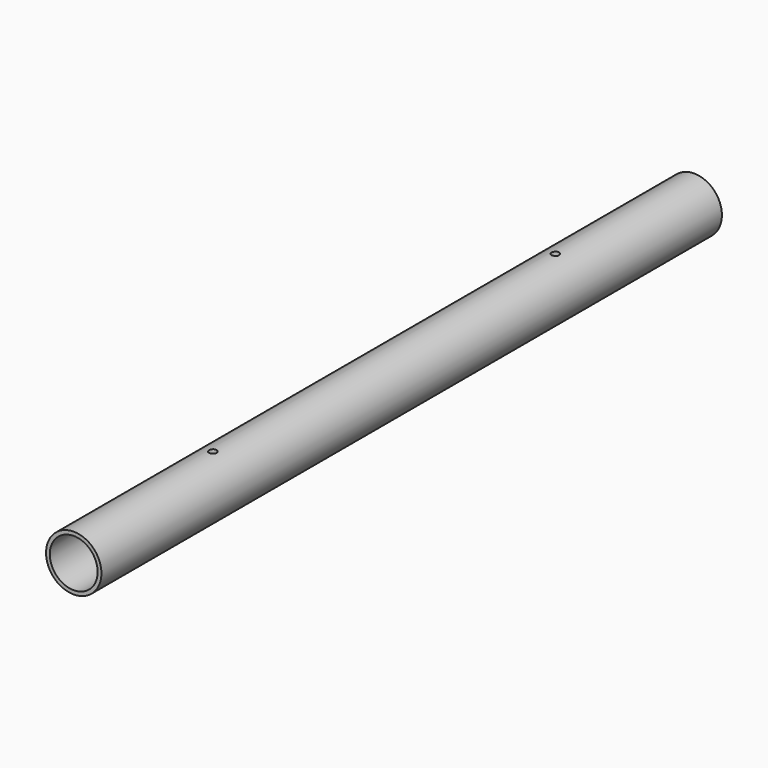
from build123d import *

# Parameters (mm, degrees)
F0_R     = 11
F0_R_2   = 9.5
F1_DEPTH = 154
F2_R     = 1.5
F3_DEPTH = 12.5


# Not quite as in the source:
# - a pattern or mirror of a feature is missing from the dataset's text; its kind, count and spacing are read off the source's solid


with BuildPart() as f1:
    # F0 (on Front) → F1 (new body, symmetric)
    with BuildSketch(Plane.XZ):
        Circle(F0_R)
        Circle(F0_R_2, mode=Mode.SUBTRACT)
    extrude(amount=F1_DEPTH, both=True)

    # F2 (on Top) → F3 (cut, symmetric)
    with BuildSketch(Plane.XY):
        with Locations((0, -85)):
            Circle(F2_R)
    f3 = extrude(amount=F3_DEPTH, both=True, mode=Mode.SUBTRACT)

    # F3_copies: F3 across plane
    add(f3.mirror(Plane.ZX), mode=Mode.SUBTRACT)


solid = f1.part
